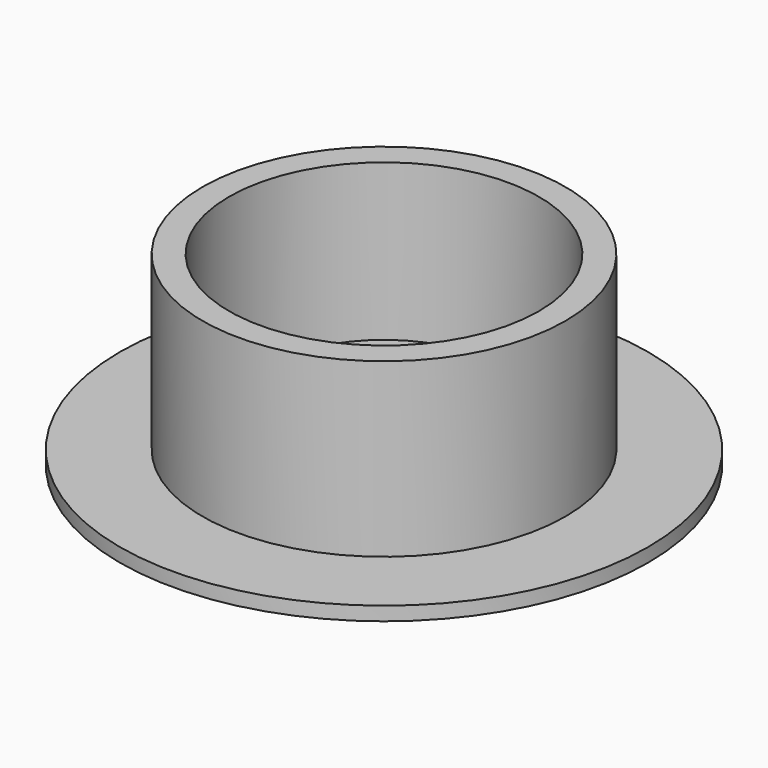
from build123d import *

# Parameters (mm, degrees)
F0_R      = 26.35
F0_R_2    = 22.5
F1_DEPTH  = 25
F2_R      = 38.35
F2_R_2    = 26.35
F2_R_3    = 22.5
F3_DEPTH  = 2
F4_R      = 11
F5_DEPTH  = 25
F6_R      = 17.3263528998
F7_DEPTH  = 5
F8_R      = 11
F9_DEPTH  = 25
F10_W     = 19.7272742478
F10_H     = 3
F10_W_2   = 21.5454568693
F11_DEPTH = 1


with BuildPart() as f1:
    # F0 (on Top) → F1 (new body)
    with BuildSketch(Plane.XY):
        Circle(F0_R)
        Circle(F0_R_2, mode=Mode.SUBTRACT)
    extrude(amount=F1_DEPTH)

    # F2 (on face) → F3 (join)
    with BuildSketch(Plane(origin=(0, 0, 0), x_dir=(1, 0, 0), z_dir=(0, 0, -1))):
        Circle(F2_R)
        Circle(F2_R_2, mode=Mode.SUBTRACT)
        Circle(F2_R_2)
        Circle(F2_R_3, mode=Mode.SUBTRACT)
        Circle(F2_R_3)
    extrude(amount=F3_DEPTH)

    # F4 (on face) → F5 (cut)
    with BuildSketch(Plane(origin=(0, 0, -2), x_dir=(1, 0, 0), z_dir=(0, 0, -1))):
        Circle(F4_R)
    extrude(amount=-F5_DEPTH, mode=Mode.SUBTRACT)

    # F6 (on face) → F7 (join)
    with BuildSketch(Plane.XY):
        Circle(F6_R)
    extrude(amount=F7_DEPTH)

    # F8 (on face) → F9 (cut)
    with BuildSketch(Plane(origin=(0, 0, 0), x_dir=(1, 0, 0), z_dir=(0, 0, -1))):
        Circle(F8_R)
    extrude(amount=-F9_DEPTH, mode=Mode.SUBTRACT)

    # F10 (on face) → F11 (join)
    with BuildSketch(Plane.XY.offset(5)):
        with Locations((0.8293200467, 10)):
            Rectangle(F10_W, F10_H)
        with Locations((0.4202285782, -10)):
            Rectangle(F10_W_2, F10_H)
    extrude(amount=-F11_DEPTH)


solid = f1.part
